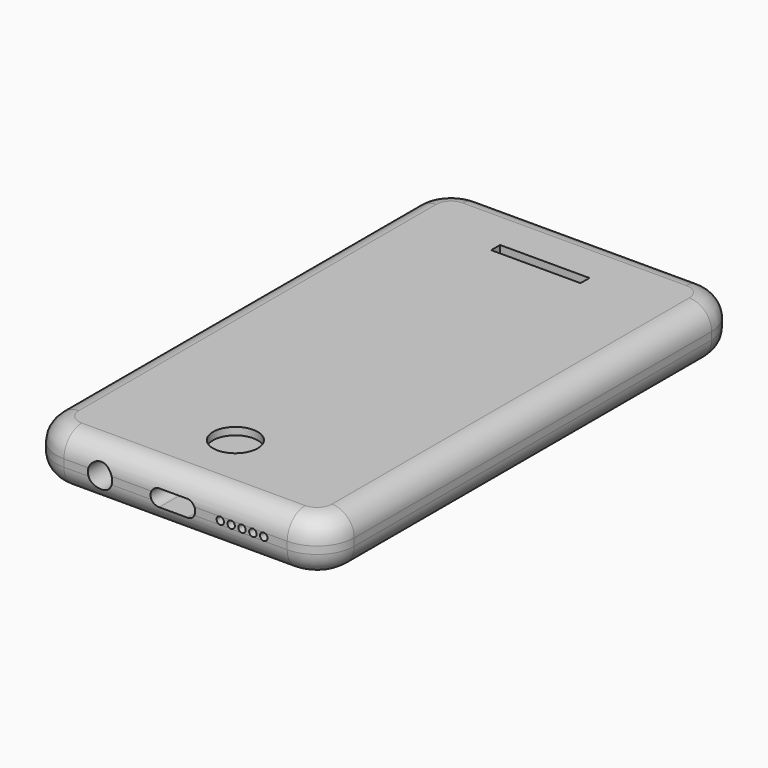
from build123d import *

# Parameters (mm, degrees)
F0_W         = 40
F0_H         = 70
F1_DEPTH     = 7
F2_R         = 5
F3_R         = 0.4991012629
F3_R_2       = 1.6336823689
F4_DEPTH     = 5
F5_T1_DEPTH  = 60
F5_T3_DEPTH  = 30
F5_T6_ANGLE  = 90
F5_T8_ANGLE  = 90
F5_T10_ANGLE = 90
F5_T12_ANGLE = 90
F5_T14_ANGLE = 90
F5_T16_ANGLE = 90
F5_T18_ANGLE = 90
F5_T20_ANGLE = 90
F6_R         = 3
F6_W         = 12
F6_H         = 1.5
F7_DEPTH     = 1


# Not quite as in the source:
# - a fillet or chamfer that OpenCascade refuses, or shapes differently, is made with other operations: its cross-section is extruded or revolved along the edge and cut away or added


with BuildPart() as f1:
    # F0 (on Top) → F1 (new body)
    with BuildSketch(Plane.XY):
        with Locations((20, 35)):
            Rectangle(F0_W, F0_H)
    extrude(amount=F1_DEPTH)

    # F2
    f2_edges = [f1.edges().sort_by_distance(p)[0] for p in [
        (40, 0, 3.5),
        (0, 0, 3.5),
        (40, 70, 3.5),
        (0, 70, 3.5),
    ]]
    fillet(f2_edges, radius=F2_R)

    # F3 (on face) → F4 (cut)
    with BuildSketch(Plane.XZ):
        with BuildLine():
            Line((21.5274822088, 4.6158107299), (17.7544243634, 4.6158107708))
            ThreePointArc((17.7544243634, 4.6158107708), (16.6386135926, 3.5), (17.7544243634, 2.3841892292))
            Line((17.7544243634, 2.3841892292), (21.5274822088, 2.3841892701))
            ThreePointArc((21.5274822088, 2.3841892701), (22.6432929266, 3.5), (21.5274822088, 4.6158107299))
        make_face()
        with Locations((26.0051637888, 3.5)):
            Circle(F3_R)
        with Locations((27.4651637888, 3.5)):
            Circle(F3_R)
        with Locations((28.9251637888, 3.5)):
            Circle(F3_R)
        with Locations((30.3851637888, 3.5)):
            Circle(F3_R)
        with Locations((31.8451637888, 3.5)):
            Circle(F3_R)
        with Locations((9.854494594, 3.5)):
            Circle(F3_R_2)
    extrude(amount=-F4_DEPTH, mode=Mode.SUBTRACT)

    # F5: fillet of radius 3 on 16 edges, made by hand

    # F5_s2 → F5_t1 (cut)
    with BuildSketch(Plane.XZ.offset(-65)):
        with BuildLine():
            ThreePointArc((0, 4), (0.8786796564, 6.1213203436), (3, 7))
            Line((3, 7), (0, 7))
            Line((0, 7), (0, 4))
        make_face()
        with BuildLine():
            ThreePointArc((0, 3), (0.8786796564, 0.8786796564), (3, 0))
            Line((3, 0), (0, 0))
            Line((0, 0), (0, 3))
        make_face()
        with BuildLine():
            ThreePointArc((37, 0), (39.1213203436, 0.8786796564), (40, 3))
            Line((40, 3), (40, 0))
            Line((40, 0), (37, 0))
        make_face()
        with BuildLine():
            ThreePointArc((37, 7), (39.1213203436, 6.1213203436), (40, 4))
            Line((40, 4), (40, 7))
            Line((40, 7), (37, 7))
        make_face()
    extrude(amount=F5_T1_DEPTH, mode=Mode.SUBTRACT)

    # F5_s4 → F5_t3 (cut)
    with BuildSketch(Plane.YZ.offset(5)):
        with BuildLine():
            ThreePointArc((67, 0), (69.1213203436, 0.8786796564), (70, 3))
            Line((70, 3), (70, 0))
            Line((70, 0), (67, 0))
        make_face()
        with BuildLine():
            ThreePointArc((3, 0), (0.8786796564, 0.8786796564), (0, 3))
            Line((0, 3), (0, 0))
            Line((0, 0), (3, 0))
        make_face()
        with BuildLine():
            ThreePointArc((67, 7), (69.1213203436, 6.1213203436), (70, 4))
            Line((70, 4), (70, 7))
            Line((70, 7), (67, 7))
        make_face()
        with BuildLine():
            ThreePointArc((3, 7), (0.8786796564, 6.1213203436), (0, 4))
            Line((0, 4), (0, 7))
            Line((0, 7), (3, 7))
        make_face()
    extrude(amount=F5_T3_DEPTH, mode=Mode.SUBTRACT)

    # F5_s5 → F5_t6 (revolve, cut)
    with BuildSketch(Plane.XZ.offset(-65)):
        with BuildLine():
            ThreePointArc((3, 0), (0.8786796564, 0.8786796564), (0, 3))
            Line((0, 3), (0, 0))
            Line((0, 0), (3, 0))
        make_face()
    revolve(axis=Axis((5, 65, 0), (0, 0, -1)), revolution_arc=F5_T6_ANGLE, mode=Mode.SUBTRACT)

    # F5_s7 → F5_t8 (revolve, cut)
    with BuildSketch(Plane.XZ.offset(-5)):
        with BuildLine():
            ThreePointArc((3, 0), (0.8786796564, 0.8786796564), (0, 3))
            Line((0, 3), (0, 0))
            Line((0, 0), (3, 0))
        make_face()
    revolve(axis=Axis((5, 5, 0), (0, 0, 1)), revolution_arc=F5_T8_ANGLE, mode=Mode.SUBTRACT)

    # F5_s9 → F5_t10 (revolve, cut)
    with BuildSketch(Plane.XZ.offset(-65)):
        with BuildLine():
            ThreePointArc((37, 0), (39.1213203436, 0.8786796564), (40, 3))
            Line((40, 3), (40, 0))
            Line((40, 0), (37, 0))
        make_face()
    revolve(axis=Axis((35, 65, 0), (0, 0, 1)), revolution_arc=F5_T10_ANGLE, mode=Mode.SUBTRACT)

    # F5_s11 → F5_t12 (revolve, cut)
    with BuildSketch(Plane.YZ.offset(35)):
        with BuildLine():
            ThreePointArc((3, 0), (0.8786796564, 0.8786796564), (0, 3))
            Line((0, 3), (0, 0))
            Line((0, 0), (3, 0))
        make_face()
    revolve(axis=Axis((35, 5, 0), (0, 0, 1)), revolution_arc=F5_T12_ANGLE, mode=Mode.SUBTRACT)

    # F5_s13 → F5_t14 (revolve, cut)
    with BuildSketch(Plane.XZ.offset(-65)):
        with BuildLine():
            ThreePointArc((0, 4), (0.8786796564, 6.1213203436), (3, 7))
            Line((3, 7), (0, 7))
            Line((0, 7), (0, 4))
        make_face()
    revolve(axis=Axis((5, 65, 7), (0, 0, -1)), revolution_arc=F5_T14_ANGLE, mode=Mode.SUBTRACT)

    # F5_s15 → F5_t16 (revolve, cut)
    with BuildSketch(Plane.XZ.offset(-5)):
        with BuildLine():
            ThreePointArc((0, 4), (0.8786796564, 6.1213203436), (3, 7))
            Line((3, 7), (0, 7))
            Line((0, 7), (0, 4))
        make_face()
    revolve(axis=Axis((5, 5, 7), (0, 0, 1)), revolution_arc=F5_T16_ANGLE, mode=Mode.SUBTRACT)

    # F5_s17 → F5_t18 (revolve, cut)
    with BuildSketch(Plane.XZ.offset(-65)):
        with BuildLine():
            ThreePointArc((37, 7), (39.1213203436, 6.1213203436), (40, 4))
            Line((40, 4), (40, 7))
            Line((40, 7), (37, 7))
        make_face()
    revolve(axis=Axis((35, 65, 7), (0, 0, 1)), revolution_arc=F5_T18_ANGLE, mode=Mode.SUBTRACT)

    # F5_s19 → F5_t20 (revolve, cut)
    with BuildSketch(Plane.YZ.offset(35)):
        with BuildLine():
            ThreePointArc((3, 7), (0.8786796564, 6.1213203436), (0, 4))
            Line((0, 4), (0, 7))
            Line((0, 7), (3, 7))
        make_face()
    revolve(axis=Axis((35, 5, 7), (0, 0, 1)), revolution_arc=F5_T20_ANGLE, mode=Mode.SUBTRACT)

    # F6 (on face) → F7 (cut)
    with BuildSketch(Plane.XY.offset(7)):
        with Locations((20, 10.0415023044)):
            Circle(F6_R)
        with Locations((20, 61.25)):
            Rectangle(F6_W, F6_H)
    extrude(amount=-F7_DEPTH, mode=Mode.SUBTRACT)


solid = f1.part
